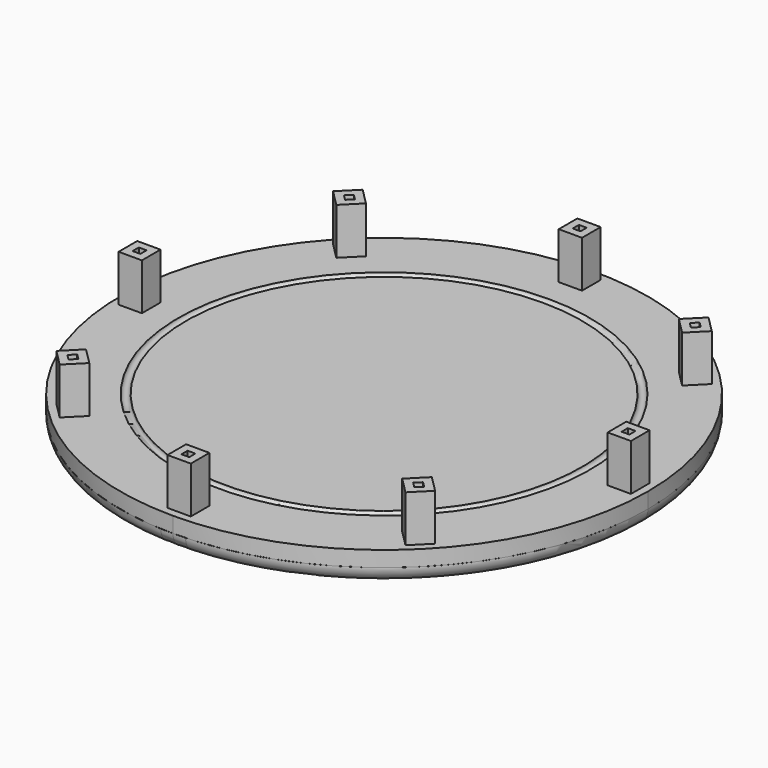
from build123d import *

# Parameters (mm, degrees)
F1_DEPTH = 5
F2_DEPTH = 20
F3_DEPTH = 10
F5_COUNT = 8
F7_DEPTH = 5
F8_R     = 4.99999


# Not quite as in the source:
# - a fillet or chamfer is up to 0.001 mm smaller than in the source, because OpenCascade refuses the exact size
# - a feature names something its author has since deleted; it is built from what else it names


with BuildPart() as f1:
    # F0 (on Top) → F1 (new body)
    with BuildSketch(Plane.XY):
        with BuildLine():
            ThreePointArc((0, -85), (60.1040764009, -60.1040764009), (85, 0))
            ThreePointArc((85, 0), (-60.1040764009, 60.1040764009), (0, -85))
        make_face()
        Polygon((3.75, -82.5), (0, -82.5), (-3.75, -82.5), (-3.75, -75), (3.75, -75), align=None, mode=Mode.SUBTRACT)
    extrude(amount=F1_DEPTH)

    # F6 (on face) + F0 (on Top) → F7 (join)
    with BuildSketch(Plane.XY):
        with BuildLine():
            ThreePointArc((85, 0), (-60.1040764009, 60.1040764009), (0, -85))
            ThreePointArc((0, -85), (60.1040764009, -60.1040764009), (85, 0))
        make_face()
        Polygon((3.75, -82.5), (0, -82.5), (-3.75, -82.5), (-3.75, -75), (3.75, -75), align=None, mode=Mode.SUBTRACT)
    with BuildSketch(Plane.XY):
        with BuildLine():
            ThreePointArc((0, -85), (60.1040764009, -60.1040764009), (85, 0))
            ThreePointArc((85, 0), (-60.1040764009, 60.1040764009), (0, -85))
        make_face()
        Polygon((3.75, -82.5), (0, -82.5), (-3.75, -82.5), (-3.75, -75), (3.75, -75), align=None, mode=Mode.SUBTRACT)
        Polygon((-3.75, -82.5), (0, -82.5), (3.75, -82.5), (3.75, -75), (-3.75, -75), align=None)
        Polygon((1.25, -80), (0, -80), (-1.25, -80), (-1.25, -77.5), (1.25, -77.5), align=None, mode=Mode.SUBTRACT)
        Polygon((-1.25, -80), (0, -80), (1.25, -80), (1.25, -77.5), (-1.25, -77.5), align=None)
    extrude(amount=-F7_DEPTH)

    # F8 (radius 5 in the source; OpenCascade refuses exactly that, so slightly less here)
    f8_edges = [f1.edges().sort_by_distance(p)[0] for p in [
        (0, 85, -5),
    ]]
    fillet(f8_edges, radius=F8_R)

    # F9 (on Right) → F10 (revolve, cut)
    with BuildSketch(Plane.YZ):
        with BuildLine():
            ThreePointArc((63.75, 5), (65, 3.75), (66.25, 5))
            ThreePointArc((66.25, 5), (65, 6.25), (63.75, 5))
        make_face()
    revolve(axis=Axis((0, 0, 2.5), (0, 0, 1)), mode=Mode.SUBTRACT)


with BuildPart() as f2:
    # F0 (on Top) → F2 (new body)
    with BuildSketch(Plane.XY):
        Polygon((-3.75, -82.5), (0, -82.5), (3.75, -82.5), (3.75, -75), (-3.75, -75), align=None)
        Polygon((1.25, -80), (0, -80), (-1.25, -80), (-1.25, -77.5), (1.25, -77.5), align=None, mode=Mode.SUBTRACT)
    extrude(amount=F2_DEPTH)

    # F0 (on Top) → F3 (join)
    with BuildSketch(Plane.XY):
        Polygon((-1.25, -80), (0, -80), (1.25, -80), (1.25, -77.5), (-1.25, -77.5), align=None)
    extrude(amount=F3_DEPTH)


with BuildPart() as f5_1:
    # F5: instance of F2
    add(f2.part.rotate(Axis((0, 0, 14.1005590558), (0, 0, 1)), 1 * 360 / F5_COUNT))


with BuildPart() as f5_2:
    # F5: instance of F2
    add(f2.part.rotate(Axis((0, 0, 14.1005590558), (0, 0, 1)), 2 * 360 / F5_COUNT))


with BuildPart() as f5_3:
    # F5: instance of F2
    add(f2.part.rotate(Axis((0, 0, 14.1005590558), (0, 0, 1)), 3 * 360 / F5_COUNT))


with BuildPart() as f5_4:
    # F5: instance of F2
    add(f2.part.rotate(Axis((0, 0, 14.1005590558), (0, 0, 1)), 4 * 360 / F5_COUNT))


with BuildPart() as f5_5:
    # F5: instance of F2
    add(f2.part.rotate(Axis((0, 0, 14.1005590558), (0, 0, 1)), 5 * 360 / F5_COUNT))


with BuildPart() as f5_6:
    # F5: instance of F2
    add(f2.part.rotate(Axis((0, 0, 14.1005590558), (0, 0, 1)), 6 * 360 / F5_COUNT))


with BuildPart() as f5_7:
    # F5: instance of F2
    add(f2.part.rotate(Axis((0, 0, 14.1005590558), (0, 0, 1)), 7 * 360 / F5_COUNT))


solid = Compound([f1.part, f2.part, f5_1.part, f5_2.part, f5_3.part, f5_4.part, f5_5.part, f5_6.part, f5_7.part])
